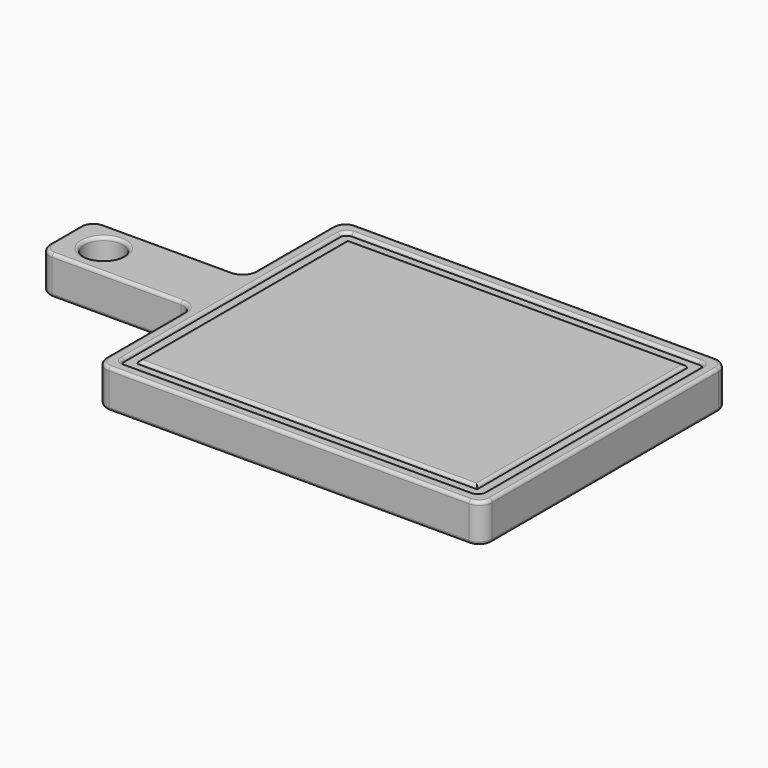
from build123d import *

# Parameters (mm, degrees)
F0_W     = 152.4
F0_H     = 63.5
F1_DEPTH = 38.1
F2_R     = 19.05
F3_DEPTH = 38.1
F5_DEPTH = 3.175
F6_R     = 6.35
F7_R     = 12.7
F8_R     = 3.17499


# Not quite as in the source:
# - a fillet or chamfer is up to 0.001 mm smaller than in the source, because OpenCascade refuses the exact size


with BuildPart() as f1:
    # F0 (on Top) → F1 (new body)
    with BuildSketch(Plane.XY):
        with Locations((-76.2, 152.4)):
            Rectangle(F0_W, F0_H)
        Polygon((0, 120.65), (0, 0), (381, 0), (381, 304.8), (0, 304.8), (0, 184.15), align=None)
    extrude(amount=F1_DEPTH)

    # F2 (on face) → F3 (cut)
    with BuildSketch(Plane(origin=(0, 0, 0), x_dir=(1, 0, 0), z_dir=(0, 0, -1))):
        with Locations((-114.3, -152.4)):
            Circle(F2_R)
    extrude(amount=-F3_DEPTH, mode=Mode.SUBTRACT)

    # F4 (on face) → F5 (cut)
    with BuildSketch(Plane.XY.offset(38.1)):
        Polygon((12.6999876976, 120.65), (12.6999876976, 12.6999876976), (368.3000123024, 12.6999876976), (368.3000123024, 292.1000123024), (12.6999876976, 292.1000123024), (12.6999876976, 184.15), align=None)
        Polygon((22.8599868298, 120.65), (22.8599868298, 184.15), (22.8599868298, 281.9400131702), (358.1400131702, 281.9400131702), (358.1400131702, 22.8599868298), (22.8599868298, 22.8599868298), align=None, mode=Mode.SUBTRACT)
    extrude(amount=-F5_DEPTH, mode=Mode.SUBTRACT)

    # F6
    f6_edges = [f1.edges().sort_by_distance(p)[0] for p in [
        (12.699988, 292.100012, 36.5125),
        (368.300012, 292.100012, 36.5125),
        (368.300012, 12.699988, 36.5125),
        (12.699988, 12.699988, 36.5125),
    ]]
    fillet(f6_edges, radius=F6_R)

    # F7
    f7_edges = [f1.edges().sort_by_distance(p)[0] for p in [
        (0, 0, 19.05),
        (-152.4, 120.65, 19.05),
        (-152.4, 184.15, 19.05),
        (0, 304.8, 19.05),
        (381, 304.8, 19.05),
        (381, 0, 19.05),
        (0, 184.15, 19.05),
        (0, 120.65, 19.05),
    ]]
    fillet(f7_edges, radius=F7_R)

    # F8 (radius 3.175 in the source; OpenCascade refuses exactly that, so slightly less here)
    f8_edges = [f1.edges().sort_by_distance(p)[0] for p in [
        (190.5, 281.940013, 38.1),
        (358.140013, 152.4, 38.1),
        (190.5, 22.859987, 38.1),
        (22.859987, 152.4, 38.1),
        (-76.2, 120.65, 38.1),
        (-148.680256, 124.369744, 38.1),
        (-3.719744, 116.930256, 38.1),
        (-152.4, 152.4, 38.1),
        (0, 60.325, 38.1),
        (-148.680256, 180.430256, 38.1),
        (3.719744, 3.719744, 38.1),
        (-76.2, 184.15, 38.1),
        (190.5, 0, 38.1),
        (-3.719744, 187.869744, 38.1),
        (377.280256, 3.719744, 38.1),
        (0, 244.475, 38.1),
        (381, 152.4, 38.1),
        (3.719744, 301.080256, 38.1),
        (377.280256, 301.080256, 38.1),
        (190.5, 304.8, 38.1),
        (190.5, 12.699988, 38.1),
        (14.55986, 14.55986, 38.1),
        (366.44014, 14.55986, 38.1),
        (12.699988, 152.4, 38.1),
        (368.300012, 152.4, 38.1),
        (14.55986, 290.24014, 38.1),
        (366.44014, 290.24014, 38.1),
        (190.5, 292.100012, 38.1),
        (-133.35, 152.4, 38.1),
        (-76.2, 120.65, 0),
        (-148.680256, 124.369744, 0),
        (-3.719744, 116.930256, 0),
        (-152.4, 152.4, 0),
        (0, 60.325, 0),
        (-148.680256, 180.430256, 0),
        (3.719744, 3.719744, 0),
        (-76.2, 184.15, 0),
        (190.5, 0, 0),
        (-3.719744, 187.869744, 0),
        (377.280256, 3.719744, 0),
        (0, 244.475, 0),
        (381, 152.4, 0),
        (3.719744, 301.080256, 0),
        (377.280256, 301.080256, 0),
        (190.5, 304.8, 0),
        (-133.35, 152.4, 0),
    ]]
    fillet(f8_edges, radius=F8_R)


solid = f1.part
